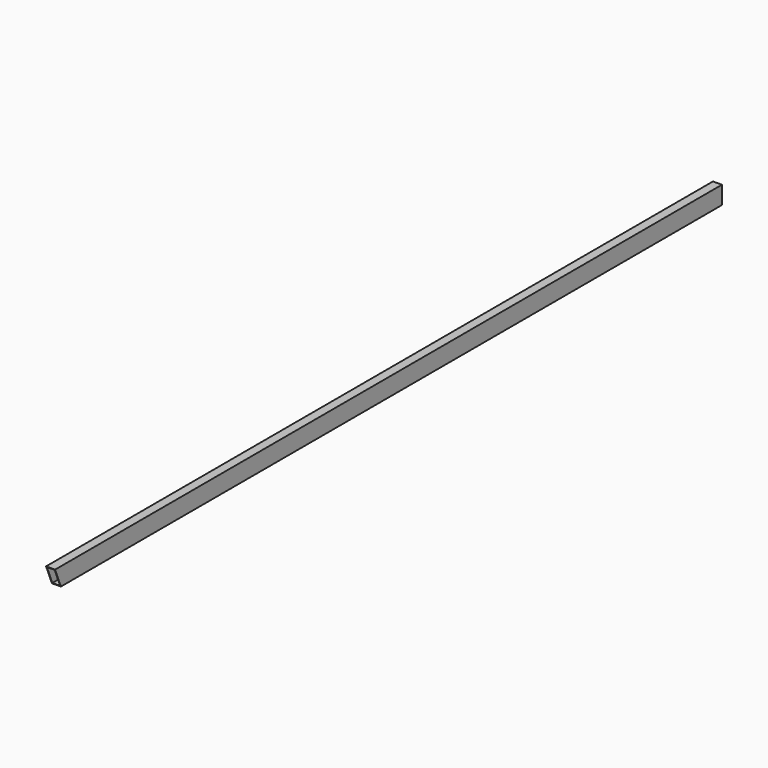
from build123d import *

# Parameters (mm, degrees)
F0_W        = 50
F0_H        = 100
F0_W_2      = 44
F0_H_2      = 94
F1_DEPTH    = 4657
F2_T1_DEPTH = 568.5605442995


# Not quite as in the source:
# - a fillet or chamfer that OpenCascade refuses, or shapes differently, is made with other operations: its cross-section is extruded or revolved along the edge and cut away or added


with BuildPart() as f1:
    # F0 (on Front) → F1 (new body)
    with BuildSketch(Plane.XZ):
        Rectangle(F0_W, F0_H)
        Rectangle(F0_W_2, F0_H_2, mode=Mode.SUBTRACT)
    extrude(amount=F1_DEPTH)

    # F2: chamfer of 41 x 100 on 1 edges, made by hand

    # F2_s2 → F2_t1 (cut)
    with BuildSketch(Plane.YZ.offset(-284.2802721497)):
        Polygon((-4616, -50), (-4657, 50), (-4657, -50), align=None)
    extrude(amount=F2_T1_DEPTH, mode=Mode.SUBTRACT)


solid = f1.part
